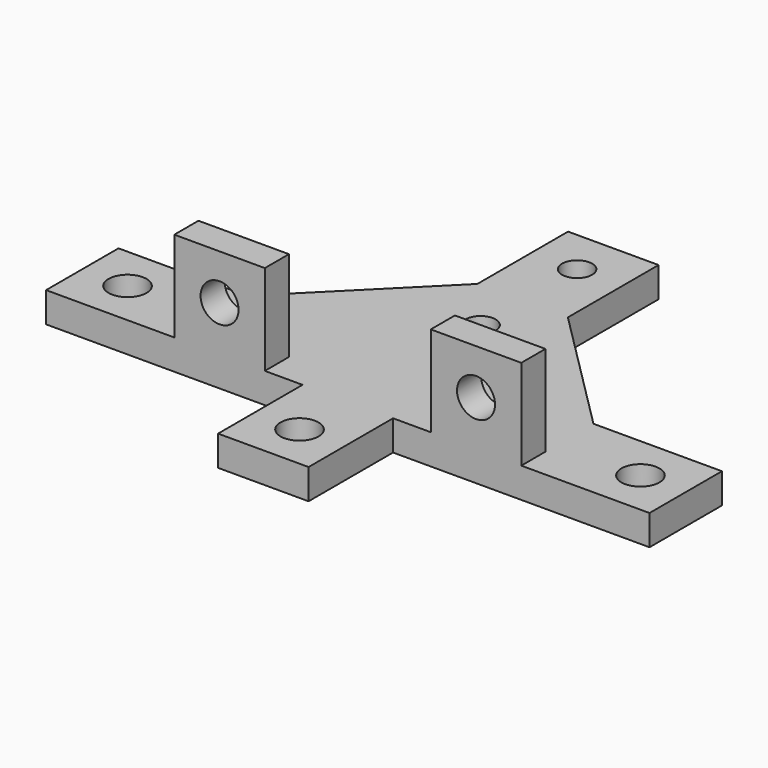
from build123d import *

# Parameters (mm, degrees)
F0_R     = 2
F0_R_2   = 1.5875
F1_DEPTH = 3.175
F2_W     = 9.525
F2_H     = 3.175
F3_DEPTH = 9.525
F4_R     = 2
F5_DEPTH = 34.926


# Not quite as in the source:
# - a length typed as a fraction of an inch, garbled in the dataset ("3 / 203.2 mm" for 3/8 in), is restored
# - a pattern or mirror of a feature is missing from the dataset's text; its kind, count and spacing are read off the source's solid


with BuildPart() as f1:
    # F0 (on Top) → F1 (new body)
    with BuildSketch(Plane.XY):
        Polygon((13.5171158184, 0), (0, 0), (0, -9.525), (26.9875, -9.525), (26.9875, -20.6375), (36.5125, -20.6375), (36.5125, -9.525), (63.5, -9.525), (63.5, 0), (49.9828841816, 0), (36.5125, 13.4703841816), (36.5125, 25.4), (26.9875, 25.4), (26.9875, 13.4703841816), align=None)
        with Locations((4.7625, -4.7625)):
            Circle(F0_R, mode=Mode.SUBTRACT)
        with Locations((31.75, -15.875)):
            Circle(F0_R, mode=Mode.SUBTRACT)
        with Locations((58.7375, -4.7625)):
            Circle(F0_R, mode=Mode.SUBTRACT)
        with Locations((31.75, 7.9375)):
            Circle(F0_R_2, mode=Mode.SUBTRACT)
        with Locations((31.75, 20.6375)):
            Circle(F0_R_2, mode=Mode.SUBTRACT)
    extrude(amount=F1_DEPTH)

    # F2 (on face) → F3 (join)
    with BuildSketch(Plane.XY.offset(3.175)):
        with Locations((18.25625, -7.9375)):
            Rectangle(F2_W, F2_H)
        with Locations((45.24375, -7.9375)):
            Rectangle(F2_W, F2_H)
    extrude(amount=F3_DEPTH)

    # F4 (on face) → F5 (cut, through all)
    with BuildSketch(Plane.XZ.offset(9.525)):
        with Locations((18.25625, 7.9375)):
            Circle(F4_R)
    f5 = extrude(amount=-F5_DEPTH, mode=Mode.SUBTRACT)

    # F5_copies: F5 across plane
    add(f5.mirror(Plane(origin=(31.75, 0, 0), x_dir=(0, 0, 1), z_dir=(1, 0, 0))), mode=Mode.SUBTRACT)


solid = f1.part
